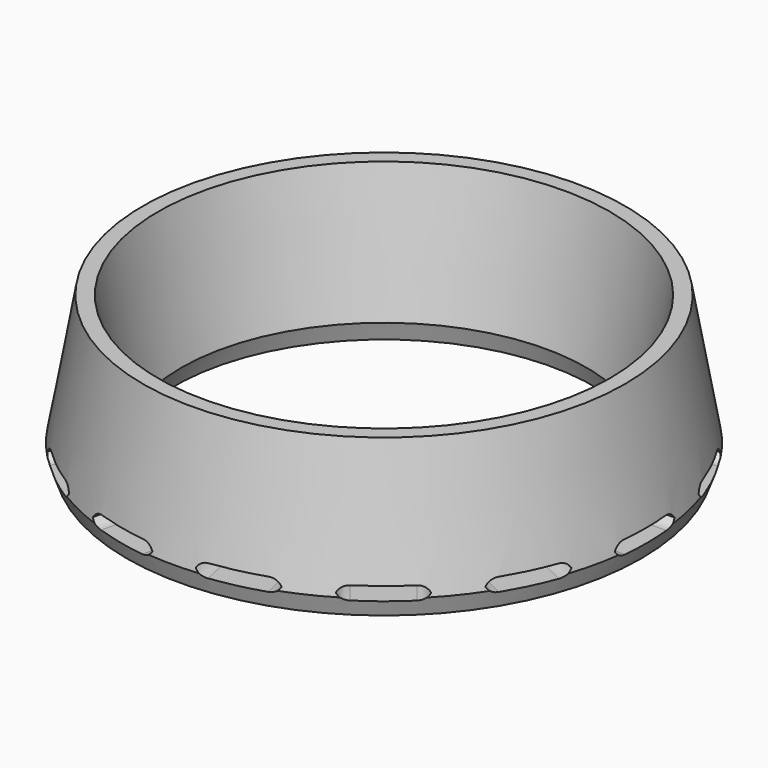
from build123d import *

# Parameters (mm, degrees)
F1_DEPTH      = 15
F2_T2_ANGLE   = 8.1362388031
F2_T4_ANGLE   = 8.1360589262
F2_T6_ANGLE   = 8.1362388031
F2_T8_ANGLE   = 8.1360589262
F3_COUNT      = 14
F4_R          = 101.5
F4_R_2        = 78.0033523804
F5_DEPTH      = 50
F5_TAPER      = 10
F5_DEPTH_BACK = 7
F5_TAPER_BACK = 20


# Not quite as in the source:
# - a fillet or chamfer that OpenCascade refuses, or shapes differently, is made with other operations: its cross-section is extruded or revolved along the edge and cut away or added


with BuildPart() as f1:
    # F0 (on Front) → F1 (new body, symmetric)
    with BuildSketch(Plane.XZ):
        with BuildLine():
            ThreePointArc((952.9285684894, 63.9279558696), (520, 18.9458343217), (85, 3.9279558696))
            Line((85, 3.9279558696), (85, -1.0720441304))
            ThreePointArc((85, -1.0720441304), (520.3448275862, 13.9577391005), (953.6165816233, 58.9755182953))
            Line((953.6165816233, 58.9755182953), (952.9285684894, 63.9279558696))
        make_face()
    extrude(amount=F1_DEPTH, both=True)

    # F2: fillet of radius 5 on 4 edges, made by hand

    # F2_s1 → F2_t2 (revolve, cut)
    with BuildSketch(Plane(origin=(955.5794732432, 0, 134.6838827396), x_dir=(0, 1, 0), z_dir=(0.9902128727, 0, 0.1395652776))):
        with BuildLine():
            ThreePointArc((-15, -74.705841471), (-13.5355339059, -71.1703075651), (-10, -69.705841471))
            Line((-10, -69.705841471), (-15, -69.705841471))
            Line((-15, -69.705841471), (-15, -74.705841471))
        make_face()
    revolve(axis=Axis((85, -15, 6311.4279558697), (0, 1, 0)), revolution_arc=F2_T2_ANGLE, mode=Mode.SUBTRACT)

    # F2_s3 → F2_t4 (revolve, cut)
    with BuildSketch(Plane(origin=(72.5017834672, 0, -0.143568521), x_dir=(0, 1, 0), z_dir=(-0.9999980394, 0, 0.0019802029))):
        with BuildLine():
            ThreePointArc((-10, 0.9161010952), (-13.5355339059, -0.5483649989), (-15, -4.0838989048))
            Line((-15, -4.0838989048), (-15, 0.9161010952))
            Line((-15, 0.9161010952), (-10, 0.9161010952))
        make_face()
    revolve(axis=Axis((85, -15, 6311.4279558698), (0, -1, 0)), revolution_arc=F2_T4_ANGLE, mode=Mode.SUBTRACT)

    # F2_s5 → F2_t6 (revolve, cut)
    with BuildSketch(Plane(origin=(955.5794732432, 0, 134.6838827396), x_dir=(0, 1, 0), z_dir=(0.9902128727, 0, 0.1395652776))):
        with BuildLine():
            ThreePointArc((10, -69.705841471), (13.5355339059, -71.1703075651), (15, -74.705841471))
            Line((15, -74.705841471), (15, -69.705841471))
            Line((15, -69.705841471), (10, -69.705841471))
        make_face()
    revolve(axis=Axis((85, 15, 6311.4279558697), (0, 1, 0)), revolution_arc=F2_T6_ANGLE, mode=Mode.SUBTRACT)

    # F2_s7 → F2_t8 (revolve, cut)
    with BuildSketch(Plane(origin=(72.5017834672, 0, -0.143568521), x_dir=(0, 1, 0), z_dir=(-0.9999980394, 0, 0.0019802029))):
        with BuildLine():
            ThreePointArc((10, 0.9161010952), (13.5355339059, -0.5483649989), (15, -4.0838989048))
            Line((15, -4.0838989048), (15, 0.9161010952))
            Line((15, 0.9161010952), (10, 0.9161010952))
        make_face()
    revolve(axis=Axis((85, 15, 6311.4279558698), (0, -1, 0)), revolution_arc=F2_T8_ANGLE, mode=Mode.SUBTRACT)


with BuildPart() as f3_1:
    # F3: instance of F1
    add(f1.part.rotate(Axis((0, 0, 116.969413124), (0, 0, 1)), 1 * 360 / F3_COUNT))


with BuildPart() as f3_2:
    # F3: instance of F1
    add(f1.part.rotate(Axis((0, 0, 116.969413124), (0, 0, 1)), 2 * 360 / F3_COUNT))


with BuildPart() as f3_3:
    # F3: instance of F1
    add(f1.part.rotate(Axis((0, 0, 116.969413124), (0, 0, 1)), 3 * 360 / F3_COUNT))


with BuildPart() as f3_4:
    # F3: instance of F1
    add(f1.part.rotate(Axis((0, 0, 116.969413124), (0, 0, 1)), 4 * 360 / F3_COUNT))


with BuildPart() as f3_5:
    # F3: instance of F1
    add(f1.part.rotate(Axis((0, 0, 116.969413124), (0, 0, 1)), 5 * 360 / F3_COUNT))


with BuildPart() as f3_6:
    # F3: instance of F1
    add(f1.part.rotate(Axis((0, 0, 116.969413124), (0, 0, 1)), 6 * 360 / F3_COUNT))


with BuildPart() as f3_7:
    # F3: instance of F1
    add(f1.part.rotate(Axis((0, 0, 116.969413124), (0, 0, 1)), 7 * 360 / F3_COUNT))


with BuildPart() as f3_8:
    # F3: instance of F1
    add(f1.part.rotate(Axis((0, 0, 116.969413124), (0, 0, 1)), 8 * 360 / F3_COUNT))


with BuildPart() as f3_9:
    # F3: instance of F1
    add(f1.part.rotate(Axis((0, 0, 116.969413124), (0, 0, 1)), 9 * 360 / F3_COUNT))


with BuildPart() as f3_10:
    # F3: instance of F1
    add(f1.part.rotate(Axis((0, 0, 116.969413124), (0, 0, 1)), 10 * 360 / F3_COUNT))


with BuildPart() as f3_11:
    # F3: instance of F1
    add(f1.part.rotate(Axis((0, 0, 116.969413124), (0, 0, 1)), 11 * 360 / F3_COUNT))


with BuildPart() as f3_12:
    # F3: instance of F1
    add(f1.part.rotate(Axis((0, 0, 116.969413124), (0, 0, 1)), 12 * 360 / F3_COUNT))


with BuildPart() as f3_13:
    # F3: instance of F1
    add(f1.part.rotate(Axis((0, 0, 116.969413124), (0, 0, 1)), 13 * 360 / F3_COUNT))


with BuildPart() as f5:
    # F4 (on Top) → F5 (new body, two sides)
    with BuildSketch(Plane.XY) as f5_sk:
        Circle(F4_R)
        Circle(F4_R_2, mode=Mode.SUBTRACT)
    extrude(amount=F5_DEPTH, taper=F5_TAPER)
    extrude(f5_sk.sketch, amount=-F5_DEPTH_BACK, taper=F5_TAPER_BACK)

    # F6: cut F1, F3_1, F3_2, F3_3, F3_4, F3_5, F3_6, F3_7, F3_8, F3_9, F3_10, F3_11, F3_12, F3_13
    add(f1.part, mode=Mode.SUBTRACT)
    add(f3_1.part, mode=Mode.SUBTRACT)
    add(f3_2.part, mode=Mode.SUBTRACT)
    add(f3_3.part, mode=Mode.SUBTRACT)
    add(f3_4.part, mode=Mode.SUBTRACT)
    add(f3_5.part, mode=Mode.SUBTRACT)
    add(f3_6.part, mode=Mode.SUBTRACT)
    add(f3_7.part, mode=Mode.SUBTRACT)
    add(f3_8.part, mode=Mode.SUBTRACT)
    add(f3_9.part, mode=Mode.SUBTRACT)
    add(f3_10.part, mode=Mode.SUBTRACT)
    add(f3_11.part, mode=Mode.SUBTRACT)
    add(f3_12.part, mode=Mode.SUBTRACT)
    add(f3_13.part, mode=Mode.SUBTRACT)


solid = f5.part
